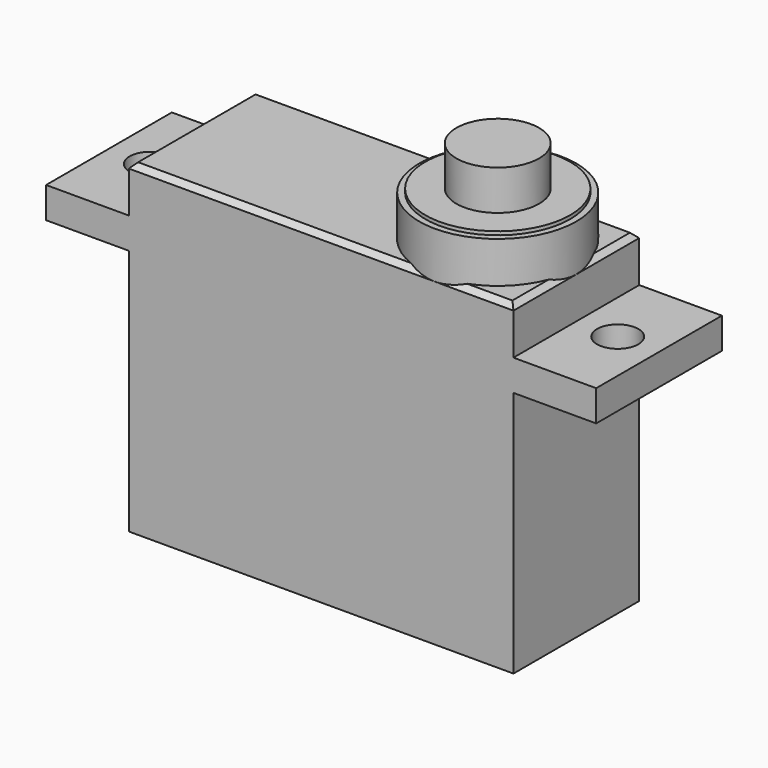
from build123d import *

# Parameters (mm, degrees)
F1_DEPTH     = 7.6
F2_R         = 1
F3_DEPTH     = 13.451
F4_R         = 3.8
F4_R_2       = 3.5
F4_R_3       = 2
F5_DEPTH     = 2
F6_DEPTH     = 2.17
F7_DEPTH     = 4.1
F8_T1_DEPTH  = 8.885841494
F8_T6_DEPTH  = 15.442920747
F8_S7_R      = 3.8
F8_T8_DEPTH  = 9
F8_T12_DEPTH = 15.442920747
F8_S13_R     = 3.8
F8_T14_DEPTH = 9
F8_T18_DEPTH = 4.442920747
F8_S19_R     = 3.8
F8_T20_DEPTH = 4
F8_T24_DEPTH = 4.442920747
F8_S25_R     = 3.8
F8_T26_DEPTH = 4
F8_T30_DEPTH = 4.442920747
F8_S31_R     = 3.8
F8_T32_DEPTH = 4
F8_T36_DEPTH = 4.442920747
F8_S37_R     = 3.8
F8_T38_DEPTH = 4


# Not quite as in the source:
# - a fillet or chamfer that OpenCascade refuses, or shapes differently, is made with other operations: its cross-section is extruded or revolved along the edge and cut away or added


with BuildPart() as f1:
    # F0 (on Front) → F1 (new body)
    with BuildSketch(Plane.XZ):
        Polygon((9.3, 15.7), (-9.3, 15.7), (-9.3, 13.45), (-13.3, 13.45), (-13.3, 11.95), (-9.3, 11.95), (-9.3, 0), (9.3, 0), (9.3, 11.95), (13.3, 11.95), (13.3, 13.45), (9.3, 13.45), align=None)
    extrude(amount=F1_DEPTH)

    # F2 (on face) → F3 (cut, through all)
    with BuildSketch(Plane.XY.offset(13.45)):
        with Locations((-11.3, -3.8)):
            Circle(F2_R)
        with Locations((11.3, -3.8)):
            Circle(F2_R)
    extrude(amount=-F3_DEPTH, mode=Mode.SUBTRACT)

    # F4 (on face) → F5 (join)
    with BuildSketch(Plane.XY.offset(15.7)):
        with Locations((5.5, -3.8)):
            Circle(F4_R)
        with Locations((5.5, -3.8)):
            Circle(F4_R_2, mode=Mode.SUBTRACT)
        with Locations((5.5, -3.8)):
            Circle(F4_R_2)
        with Locations((5.5, -3.8)):
            Circle(F4_R_3, mode=Mode.SUBTRACT)
        with Locations((5.5, -3.8)):
            Circle(F4_R_3)
    extrude(amount=F5_DEPTH)

    # F4 (on face) → F6 (join)
    with BuildSketch(Plane.XY.offset(15.7)):
        with Locations((5.5, -3.8)):
            Circle(F4_R_2)
        with Locations((5.5, -3.8)):
            Circle(F4_R_3, mode=Mode.SUBTRACT)
        with Locations((5.5, -3.8)):
            Circle(F4_R_3)
    extrude(amount=F6_DEPTH)

    # F4 (on face) → F7 (join)
    with BuildSketch(Plane.XY.offset(15.7)):
        with Locations((5.5, -3.8)):
            Circle(F4_R_3)
    extrude(amount=F7_DEPTH)

    # F8: chamfer of 0.25 on 7 edges, made by hand

    # F8_s2 → F8_t1 (cut)
    with BuildSketch(Plane.XZ.offset(-0.642920747)):
        Polygon((-9.05, 15.7), (-9.3, 15.45), (-9.3, 15.7), align=None)
    extrude(amount=F8_T1_DEPTH, mode=Mode.SUBTRACT)


with BuildPart() as f8_tool4:
    # F8_s5 → F8_t6 (new body)
    with BuildSketch(Plane.YZ.offset(5.5)):
        Polygon((-7.35, 15.7), (-7.6, 15.45), (-7.6, 15.7), align=None)
    extrude(amount=-F8_T6_DEPTH)

    # F8_s7 → F8_t8 (cut, symmetric)
    with BuildSketch(Plane.XY.offset(15.6)):
        with Locations((5.5, -3.8)):
            Circle(F8_S7_R)
    extrude(amount=F8_T8_DEPTH, both=True, mode=Mode.SUBTRACT)


with BuildPart() as f1_1:
    add(f1.part)

    # F8_t3: cut F8_tool4
    add(f8_tool4.part, mode=Mode.SUBTRACT)


with BuildPart() as f8_tool10:
    # F8_s11 → F8_t12 (new body)
    with BuildSketch(Plane.YZ.offset(5.5)):
        Polygon((0, 15.45), (-0.25, 15.7), (0, 15.7), align=None)
    extrude(amount=-F8_T12_DEPTH)

    # F8_s13 → F8_t14 (cut, symmetric)
    with BuildSketch(Plane.XY.offset(15.6)):
        with Locations((5.5, -3.8)):
            Circle(F8_S13_R)
    extrude(amount=F8_T14_DEPTH, both=True, mode=Mode.SUBTRACT)


with BuildPart() as f1_2:
    add(f1_1.part)

    # F8_t9: cut F8_tool10
    add(f8_tool10.part, mode=Mode.SUBTRACT)


with BuildPart() as f8_tool16:
    # F8_s17 → F8_t18 (new body)
    with BuildSketch(Plane.XZ.offset(3.8)):
        Polygon((9.3, 15.45), (9.05, 15.7), (9.3, 15.7), align=None)
    extrude(amount=F8_T18_DEPTH)

    # F8_s19 → F8_t20 (cut, symmetric)
    with BuildSketch(Plane.XY.offset(15.6)):
        with Locations((5.5, -3.8)):
            Circle(F8_S19_R)
    extrude(amount=F8_T20_DEPTH, both=True, mode=Mode.SUBTRACT)


with BuildPart() as f1_3:
    add(f1_2.part)

    # F8_t15: cut F8_tool16
    add(f8_tool16.part, mode=Mode.SUBTRACT)


with BuildPart() as f8_tool22:
    # F8_s23 → F8_t24 (new body)
    with BuildSketch(Plane.YZ.offset(9.942920747)):
        Polygon((-0.25, 15.7), (0, 15.45), (0, 15.7), align=None)
    extrude(amount=-F8_T24_DEPTH)

    # F8_s25 → F8_t26 (cut, symmetric)
    with BuildSketch(Plane.XY.offset(15.6)):
        with Locations((5.5, -3.8)):
            Circle(F8_S25_R)
    extrude(amount=F8_T26_DEPTH, both=True, mode=Mode.SUBTRACT)


with BuildPart() as f1_4:
    add(f1_3.part)

    # F8_t21: cut F8_tool22
    add(f8_tool22.part, mode=Mode.SUBTRACT)


with BuildPart() as f8_tool28:
    # F8_s29 → F8_t30 (new body)
    with BuildSketch(Plane.XZ.offset(-0.642920747)):
        Polygon((9.05, 15.7), (9.3, 15.45), (9.3, 15.7), align=None)
    extrude(amount=F8_T30_DEPTH)

    # F8_s31 → F8_t32 (cut, symmetric)
    with BuildSketch(Plane.XY.offset(15.6)):
        with Locations((5.5, -3.8)):
            Circle(F8_S31_R)
    extrude(amount=F8_T32_DEPTH, both=True, mode=Mode.SUBTRACT)


with BuildPart() as f1_5:
    add(f1_4.part)

    # F8_t27: cut F8_tool28
    add(f8_tool28.part, mode=Mode.SUBTRACT)


with BuildPart() as f8_tool34:
    # F8_s35 → F8_t36 (new body)
    with BuildSketch(Plane.YZ.offset(9.942920747)):
        Polygon((-7.35, 15.7), (-7.6, 15.45), (-7.6, 15.7), align=None)
    extrude(amount=-F8_T36_DEPTH)

    # F8_s37 → F8_t38 (cut, symmetric)
    with BuildSketch(Plane.XY.offset(15.6)):
        with Locations((5.5, -3.8)):
            Circle(F8_S37_R)
    extrude(amount=F8_T38_DEPTH, both=True, mode=Mode.SUBTRACT)


with BuildPart() as f1_6:
    add(f1_5.part)

    # F8_t33: cut F8_tool34
    add(f8_tool34.part, mode=Mode.SUBTRACT)


solid = f1_6.part
